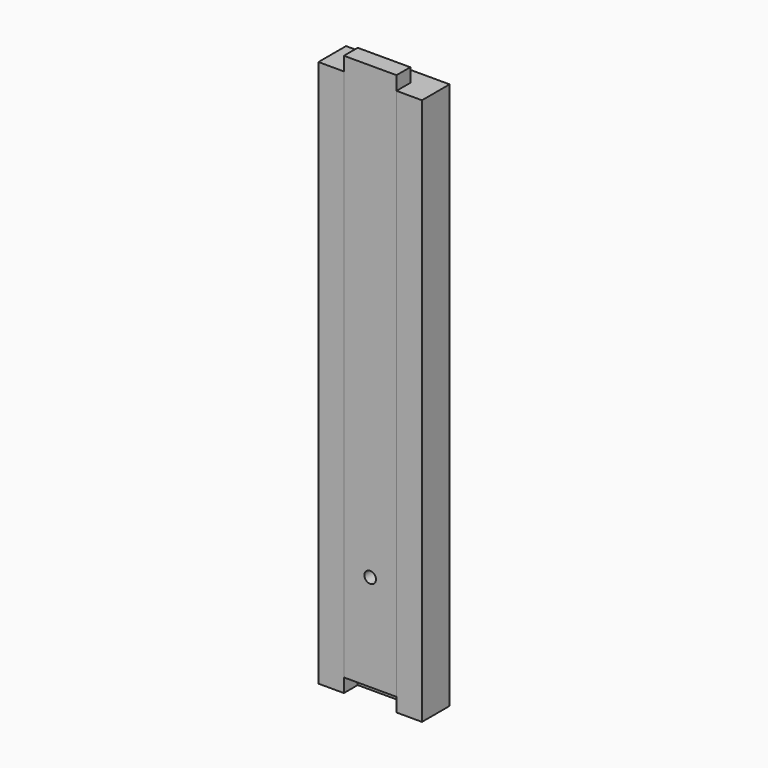
from build123d import *

# Parameters (mm, degrees)
F2_DEPTH = 198.2
F3_START = 5
F1_W     = 19.05
F1_H     = 6.25
F3_DEPTH = 198.2
F4_R     = 2.0828
F5_DEPTH = 12.501
F6_R     = 2.0828
F7_DEPTH = 25


# Not quite as in the source:
# - a feature names something its author has since deleted; it is built from what else it names


with BuildPart() as f2:
    # F1 (on Top) → F2 (new body, through all)
    with BuildSketch(Plane.XY):
        Polygon((-9.225, 0), (0, 0), (0, 12.5), (-37.5, 12.5), (-37.5, 0), (-28.275, 0), (-28.275, 6.25), (-9.225, 6.25), align=None)
    extrude(amount=F2_DEPTH)

    # F6 (on face) → F7 (cut)
    with BuildSketch(Plane(origin=(0, 12.5, 0), x_dir=(-1, 0, 0), z_dir=(0, 1, 0))):
        with Locations((18.75, 142.2)):
            Circle(F6_R)
        with Locations((18.75, 172.2)):
            Circle(F6_R)
    extrude(amount=-F7_DEPTH, mode=Mode.SUBTRACT)


with BuildPart() as f3:
    # F1 (on Top) → F3 (new body)
    with BuildSketch(Plane.XY.offset(F3_START)):
        with Locations((-18.75, 3.125)):
            Rectangle(F1_W, F1_H)
    extrude(amount=F3_DEPTH)

    # F4 (on face) → F5 (cut, through all)
    with BuildSketch(Plane.XZ):
        with Locations((-18.75, 40)):
            Circle(F4_R)
    extrude(amount=-F5_DEPTH, mode=Mode.SUBTRACT)


solid = Compound([f2.part, f3.part])
